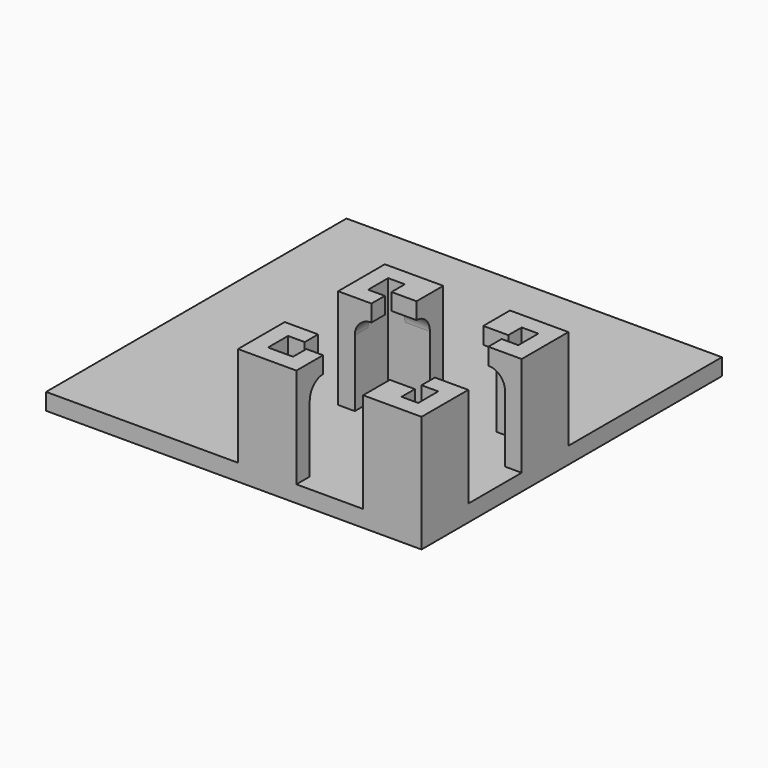
from build123d import *

# Parameters (mm, degrees)
F0_W     = 45
F0_H     = 45
F1_DEPTH = 2
F2_W     = 22
F2_H     = 22
F2_W_2   = 18
F2_H_2   = 18
F3_DEPTH = 10
F4_W     = 22
F4_H     = 22
F4_W_2   = 2
F4_H_2   = 12
F4_W_3   = 14
F4_H_3   = 2
F4_W_4   = 13
F5_DEPTH = 2
F6_R     = 1.99999
F7_W     = 11
F7_H     = 8
F7_W_2   = 8
F7_H_2   = 11
F8_DEPTH = 12


# Not quite as in the source:
# - a fillet or chamfer is up to 0.001 mm smaller than in the source, because OpenCascade refuses the exact size


with BuildPart() as f1:
    # F0 (on Top) → F1 (new body)
    with BuildSketch(Plane.XY):
        with Locations((22.5, -22.5)):
            Rectangle(F0_W, F0_H)
    extrude(amount=F1_DEPTH)

    # F2 (on face) → F3 (join)
    with BuildSketch(Plane.XY.offset(2)):
        with Locations((34, -34)):
            Rectangle(F2_W, F2_H)
        with Locations((34, -34)):
            Rectangle(F2_W_2, F2_H_2, mode=Mode.SUBTRACT)
    extrude(amount=F3_DEPTH)

    # F4 (on face) → F5 (join)
    with BuildSketch(Plane.XY.offset(12)):
        with Locations((34, -34)):
            Rectangle(F4_W, F4_H)
        Polygon((28, -43), (25, -43), (25, -40), (25, -28), (25, -25), (27, -25), (41, -25), (43, -25), (43, -28), (43, -40), (43, -43), (41, -43), align=None, mode=Mode.SUBTRACT)
        with Locations((26, -34)):
            Rectangle(F4_W_2, F4_H_2)
        with Locations((34, -26)):
            Rectangle(F4_W_3, F4_H_3)
        with Locations((42, -34)):
            Rectangle(F4_W_2, F4_H_2)
        with Locations((34.5, -42)):
            Rectangle(F4_W_4, F4_H_3)
    extrude(amount=F5_DEPTH)

    # F6 (radius 2 in the source; OpenCascade refuses exactly that, so slightly less here)
    f6_edges = [f1.edges().sort_by_distance(p)[0] for p in [
        (25, -34, 12),
        (43, -34, 12),
        (34, -25, 12),
        (34.5, -43, 12),
    ]]
    fillet(f6_edges, radius=F6_R)

    # F7 (on face) → F8 (cut, through all)
    with BuildSketch(Plane.XY.offset(14)):
        with Locations((43.5, -34)):
            Rectangle(F7_W, F7_H)
        with Locations((34, -43.5)):
            Rectangle(F7_W_2, F7_H_2)
        with Locations((34, -34)):
            Rectangle(F7_W_2, F7_H)
        with Locations((24.5, -34)):
            Rectangle(F7_W, F7_H)
        with Locations((34, -24.5)):
            Rectangle(F7_W_2, F7_H_2)
    extrude(amount=-F8_DEPTH, mode=Mode.SUBTRACT)


solid = f1.part
